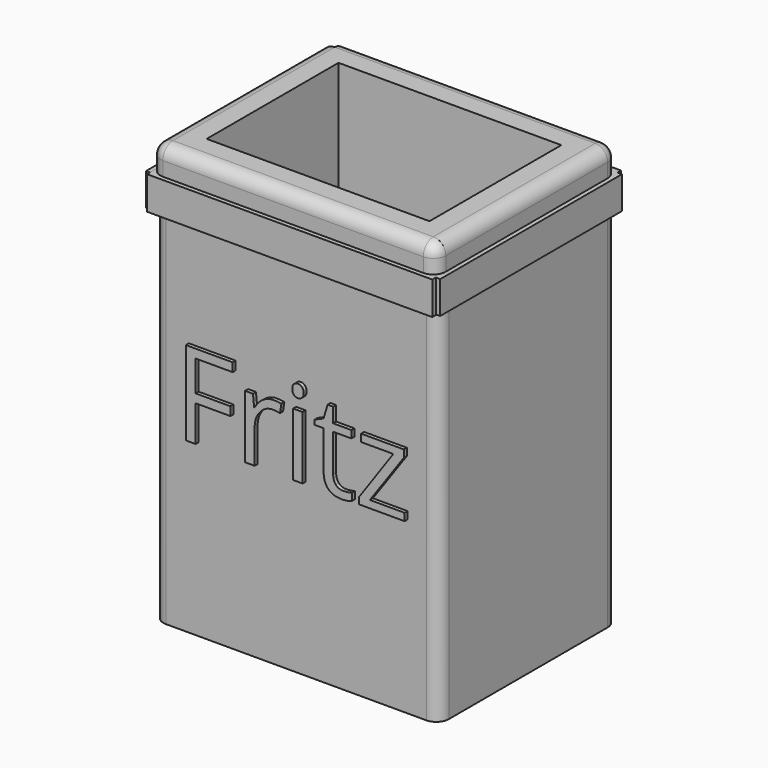
from build123d import *

# Parameters (mm, degrees)
F0_W          = 115.9102246165
F0_H          = 92.3246163875
F1_DEPTH      = 171.45
F2_T          = -12.7
F3_R          = 5.08
F4_W          = 115.9102246165
F4_H          = 13.2569223642
F6_DEPTH      = 1.778
F5_W          = 92.3246163875
F5_H          = 13.2491886616
F7_DEPTH      = 1.778
F8_W          = 92.3246163875
F8_H          = 13.2032483816
F9_DEPTH      = 1.778
F11_DEPTH     = 1.778
F12_W         = 115.9102246165
F12_H         = 147.1718251705
F12_W_2       = 3.8736611168
F12_H_2       = 25.5631778903
F13_DEPTH     = 1.524
F14_R         = 5.08
F15_T1_DEPTH  = 5.7646141005
F15_S5_W      = 5.08
F15_S5_H      = 5.08
F15_T6_DEPTH  = 5.08
F15_S11_W     = 5.08
F15_S11_H     = 5.08
F15_T12_DEPTH = 5.08
F15_S17_W     = 5.08
F15_S17_H     = 5.08
F15_T18_DEPTH = 5.08
F15_S23_W     = 5.08
F15_S23_H     = 5.08
F15_T24_DEPTH = 5.08


# Not quite as in the source:
# - a fillet or chamfer that OpenCascade refuses, or shapes differently, is made with other operations: its cross-section is extruded or revolved along the edge and cut away or added
# - a feature names something its author has since deleted; it is built from what else it names


with BuildPart() as f1:
    # F0 (on Top) → F1 (new body)
    with BuildSketch(Plane.XY):
        with Locations((2.3365281522, -22.1691494808)):
            Rectangle(F0_W, F0_H)
    extrude(amount=F1_DEPTH)

    # F2
    f2_openings = [f1.faces().sort_by_distance(p)[0] for p in [
        (2.336528, -22.169149, 171.45),
    ]]
    offset(amount=F2_T, openings=f2_openings)

    # F3
    f3_edges = [f1.edges().sort_by_distance(p)[0] for p in [
        (60.29164, -22.169149, 171.45),
        (2.336528, 23.993159, 171.45),
        (-55.618584, -22.169149, 171.45),
        (2.336528, -68.331458, 171.45),
    ]]
    fillet(f3_edges, radius=F3_R)

    # F4 (on face) → F6 (join)
    with BuildSketch(Plane(origin=(0, 23.993158713, 0), x_dir=(-1, 0, 0), z_dir=(0, 1, 0))):
        with Locations((-2.3365281522, 153.9769247174)):
            Rectangle(F4_W, F4_H)
    extrude(amount=F6_DEPTH)

    # F5 (on face) → F7 (join)
    with BuildSketch(Plane(origin=(-55.618584156, 0, 0), x_dir=(0, -1, 0), z_dir=(-1, 0, 0))):
        with Locations((22.1691494808, 153.7964195013)):
            Rectangle(F5_W, F5_H)
    extrude(amount=F7_DEPTH)

    # F8 (on face) → F9 (join)
    with BuildSketch(Plane.YZ.offset(60.2916404605)):
        with Locations((-22.1691494808, 154.0037617087)):
            Rectangle(F8_W, F8_H)
    extrude(amount=F9_DEPTH)

    # F10 (on face) → F11 (join)
    with BuildSketch(Plane.XZ.offset(68.3314576745)):
        Polygon((60.2916404605, 147.4021375179), (60.2916404605, 160.6053858995), (-55.618584156, 160.6053858995), (-55.618584156, 160.4210138321), (-55.618584156, 147.1718251705), (60.2916404605, 147.1718251705), align=None)
    extrude(amount=F11_DEPTH)

    # F12 (on face) → F13 (cut)
    with BuildSketch(Plane.XZ.offset(68.3314576745)):
        with Locations((2.3365281522, 73.5859125853)):
            Rectangle(F12_W, F12_H)
        Polygon((-37.2516920373, 83.9250860008), (-37.2516920373, 69.3484768271), (-41.214917573, 69.3484768271), (-41.214917573, 103.4501293179), (-22.2048696645, 103.4501293179), (-22.2048696645, 99.9272621751), (-37.2516920373, 99.9272621751), (-37.2516920373, 87.4479531437), (-23.1154412565, 87.4479531437), (-23.1154412565, 83.9250860008), align=None, mode=Mode.SUBTRACT)
        with BuildLine():
            add(Edge.make_bspline(
                [(-9.8897620677, 94.027206081), (-7.8820263443, 95.3818679166), (-5.4787144375, 95.3818679166)],
                knots=[0, 0, 0, 1, 1, 1], degree=2))
            add(Edge.make_bspline(
                [(-5.4787144375, 95.3818679166), (-3.7769904787, 95.3818679166), (-2.4260604938, 95.0982472568)],
                knots=[0, 0, 0, 1, 1, 1], degree=2))
            Line((-2.4260604938, 95.0982472568), (-2.9634470072, 91.5082067998))
            add(Edge.make_bspline(
                [(-2.9634470072, 91.5082067998), (-4.5457517408, 91.8590007738), (-5.7623350973, 91.8590007738)],
                knots=[0, 0, 0, 1, 1, 1], degree=2))
            add(Edge.make_bspline(
                [(-5.7623350973, 91.8590007738), (-8.867234952, 91.8590007738), (-11.0690269163, 89.3400014926)],
                knots=[0, 0, 0, 1, 1, 1], degree=2))
            add(Edge.make_bspline(
                [(-11.0690269163, 89.3400014926), (-13.2708188806, 86.8210022115), (-13.2708188806, 83.0667603198)],
                knots=[0, 0, 0, 1, 1, 1], degree=2))
            Line((-13.2708188806, 83.0667603198), (-13.2708188806, 69.3484768271))
            Line((-13.2708188806, 69.3484768271), (-17.1444799974, 69.3484768271))
            Line((-17.1444799974, 69.3484768271), (-17.1444799974, 94.9116547175))
            Line((-17.1444799974, 94.9116547175), (-13.9500157238, 94.9116547175))
            Line((-13.9500157238, 94.9116547175), (-13.5021936294, 90.1796679197))
            Line((-13.5021936294, 90.1796679197), (-13.31560109, 90.1796679197))
            add(Edge.make_bspline(
                [(-13.31560109, 90.1796679197), (-11.897497791, 92.6725442453), (-9.8897620677, 94.027206081)],
                knots=[0, 0, 0, 1, 1, 1], degree=2))
        make_face(mode=Mode.SUBTRACT)
        with Locations((4.2950027734, 82.1300657723)):
            Rectangle(F12_W_2, F12_H_2, mode=Mode.SUBTRACT)
        with BuildLine():
            add(Edge.make_bspline(
                [(19.6888872694, 73.3154342136), (20.7860514007, 72.0801916032), (22.6967590036, 72.0801916032)],
                knots=[0, 0, 0, 1, 1, 1], degree=2))
            add(Edge.make_bspline(
                [(22.6967590036, 72.0801916032), (23.7267498208, 72.0801916032), (24.6821036223, 72.2294656346)],
                knots=[0, 0, 0, 1, 1, 1], degree=2))
            add(Edge.make_bspline(
                [(24.6821036223, 72.2294656346), (25.6374574237, 72.3787396661), (26.1972350418, 72.5429411007)],
                knots=[0, 0, 0, 1, 1, 1], degree=2))
            Line((26.1972350418, 72.5429411007), (26.1972350418, 69.5798515759))
            add(Edge.make_bspline(
                [(26.1972350418, 69.5798515759), (25.5702841096, 69.281303513), (24.3462370515, 69.0797835705)],
                knots=[0, 0, 0, 1, 1, 1], degree=2))
            add(Edge.make_bspline(
                [(24.3462370515, 69.0797835705), (23.1221899933, 68.878263628), (22.1369813856, 68.878263628)],
                knots=[0, 0, 0, 1, 1, 1], degree=2))
            add(Edge.make_bspline(
                [(22.1369813856, 68.878263628), (14.7255257228, 68.878263628), (14.7255257228, 76.6927591758)],
                knots=[0, 0, 0, 1, 1, 1], degree=2))
            Line((14.7255257228, 76.6927591758), (14.7255257228, 91.9037829832))
            Line((14.7255257228, 91.9037829832), (11.0608482501, 91.9037829832))
            Line((11.0608482501, 91.9037829832), (11.0608482501, 93.7697083767))
            Line((11.0608482501, 93.7697083767), (14.7255257228, 95.3818679166))
            Line((14.7255257228, 95.3818679166), (16.3526126659, 100.8378337671))
            Line((16.3526126659, 100.8378337671), (18.591723138, 100.8378337671))
            Line((18.591723138, 100.8378337671), (18.591723138, 94.9116547175))
            Line((18.591723138, 94.9116547175), (26.0106425024, 94.9116547175))
            Line((26.0106425024, 94.9116547175), (26.0106425024, 91.9037829832))
            Line((26.0106425024, 91.9037829832), (18.591723138, 91.9037829832))
            Line((18.591723138, 91.9037829832), (18.591723138, 76.8569606104))
            add(Edge.make_bspline(
                [(18.591723138, 76.8569606104), (18.591723138, 74.5506768241), (19.6888872694, 73.3154342136)],
                knots=[0, 0, 0, 1, 1, 1], degree=2))
        make_face(mode=Mode.SUBTRACT)
        with BuildLine():
            add(Edge.make_bspline(
                [(2.6828432334, 99.8899436672), (2.0297693457, 100.5318220026), (2.0297693457, 101.837969778)],
                knots=[0, 0, 0, 1, 1, 1], degree=2))
            add(Edge.make_bspline(
                [(2.0297693457, 101.837969778), (2.0297693457, 103.1665086581), (2.6828432334, 103.7859958888)],
                knots=[0, 0, 0, 1, 1, 1], degree=2))
            add(Edge.make_bspline(
                [(2.6828432334, 103.7859958888), (3.3359171211, 104.4054831194), (4.3211257289, 104.4054831194)],
                knots=[0, 0, 0, 1, 1, 1], degree=2))
            add(Edge.make_bspline(
                [(4.3211257289, 104.4054831194), (5.2540884256, 104.4054831194), (5.9295534181, 103.7748003364)],
                knots=[0, 0, 0, 1, 1, 1], degree=2))
            add(Edge.make_bspline(
                [(5.9295534181, 103.7748003364), (6.6050184105, 103.1441175534), (6.6050184105, 101.837969778)],
                knots=[0, 0, 0, 1, 1, 1], degree=2))
            add(Edge.make_bspline(
                [(6.6050184105, 101.837969778), (6.6050184105, 100.5318220026), (5.9295534181, 99.8899436672)],
                knots=[0, 0, 0, 1, 1, 1], degree=2))
            add(Edge.make_bspline(
                [(5.9295534181, 99.8899436672), (5.2540884256, 99.2480653319), (4.3211257289, 99.2480653319)],
                knots=[0, 0, 0, 1, 1, 1], degree=2))
            add(Edge.make_bspline(
                [(4.3211257289, 99.2480653319), (3.3359171211, 99.2480653319), (2.6828432334, 99.8899436672)],
                knots=[0, 0, 0, 1, 1, 1], degree=2))
        make_face(mode=Mode.SUBTRACT)
        Polygon((47.6553770665, 72.3563485614), (47.6553770665, 69.3484768271), (29.1080786556, 69.3484768271), (29.1080786556, 71.9831634827), (43.057736897, 91.9037829832), (29.9738680381, 91.9037829832), (29.9738680381, 94.9116547175), (47.3045830925, 94.9116547175), (47.3045830925, 91.9037829832), (33.5415173904, 72.3563485614), align=None, mode=Mode.SUBTRACT)
    extrude(amount=-F13_DEPTH, mode=Mode.SUBTRACT)

    # F14
    f14_edges = [f1.edges().sort_by_distance(p)[0] for p in [
        (60.29164, -66.807458, 73.585913),
        (-55.618584, -66.807458, 73.585913),
        (-55.618584, 23.993159, 73.585913),
        (60.29164, 23.993159, 73.674232),
    ]]
    fillet(f14_edges, radius=F14_R)

    # F15: fillet of radius 5.08 on 4 edges, made by hand

    # F15_s2 → F15_t1 (cut)
    with BuildSketch(Plane.XY.offset(160.6053858995)):
        with BuildLine():
            ThreePointArc((-55.618584156, -63.2514576745), (-54.1306866045, -66.8435601229), (-50.538584156, -68.3314576745))
            Line((-50.538584156, -68.3314576745), (-55.618584156, -68.3314576745))
            Line((-55.618584156, -68.3314576745), (-55.618584156, -63.2514576745))
        make_face()
        with BuildLine():
            ThreePointArc((55.2116404605, -68.3314576745), (58.8037429089, -66.8435601229), (60.2916404605, -63.2514576745))
            Line((60.2916404605, -63.2514576745), (60.2916404605, -68.3314576745))
            Line((60.2916404605, -68.3314576745), (55.2116404605, -68.3314576745))
        make_face()
        with BuildLine():
            ThreePointArc((55.2116404605, 23.993158713), (58.8037429089, 22.5052611614), (60.2916404605, 18.913158713))
            Line((60.2916404605, 18.913158713), (60.2916404605, 23.993158713))
            Line((60.2916404605, 23.993158713), (55.2116404605, 23.993158713))
        make_face()
        with BuildLine():
            ThreePointArc((-55.618584156, 18.913158713), (-54.1306866045, 22.5052611614), (-50.538584156, 23.993158713))
            Line((-50.538584156, 23.993158713), (-55.618584156, 23.993158713))
            Line((-55.618584156, 23.993158713), (-55.618584156, 18.913158713))
        make_face()
    extrude(amount=F15_T1_DEPTH, mode=Mode.SUBTRACT)


with BuildPart() as f15_tool4:
    # F15_s5 → F15_t6 (new body)
    with BuildSketch(Plane.YZ.offset(-50.538584156)):
        with Locations((21.453158713, 168.91)):
            Rectangle(F15_S5_W, F15_S5_H)
    extrude(amount=-F15_T6_DEPTH)

    # F15_s7 → F15_t8 (revolve, cut)
    with BuildSketch(Plane(origin=(-50.538584156, 18.913158713, 166.37), x_dir=(0, -0.7071067812, -0.7071067812), z_dir=(0, 0.7071067812, -0.7071067812))):
        with BuildLine():
            ThreePointArc((0, -5.08), (5.08, 0), (0, 5.08))
            Line((0, 5.08), (0, -5.08))
        make_face()
    revolve(axis=Axis((-50.538584156, 18.913158713, 166.37), (-1, 0, 0)), mode=Mode.SUBTRACT)


with BuildPart() as f1_1:
    add(f1.part)

    # F15_t3: cut F15_tool4
    add(f15_tool4.part, mode=Mode.SUBTRACT)


with BuildPart() as f15_tool10:
    # F15_s11 → F15_t12 (new body)
    with BuildSketch(Plane.XZ.offset(-18.913158713)):
        with Locations((57.7516404605, 168.91)):
            Rectangle(F15_S11_W, F15_S11_H)
    extrude(amount=-F15_T12_DEPTH)

    # F15_s13 → F15_t14 (revolve, cut)
    with BuildSketch(Plane(origin=(55.2116404605, 18.913158713, 166.37), x_dir=(-0.7071067812, 0, -0.7071067812), z_dir=(0.7071067812, 0, -0.7071067812))):
        with BuildLine():
            ThreePointArc((0, -5.08), (5.08, 0), (0, 5.08))
            Line((0, 5.08), (0, -5.08))
        make_face()
    revolve(axis=Axis((55.2116404605, 18.913158713, 166.37), (0, 1, 0)), mode=Mode.SUBTRACT)


with BuildPart() as f1_2:
    add(f1_1.part)

    # F15_t9: cut F15_tool10
    add(f15_tool10.part, mode=Mode.SUBTRACT)


with BuildPart() as f15_tool16:
    # F15_s17 → F15_t18 (new body)
    with BuildSketch(Plane.XZ.offset(63.2514576745)):
        with Locations((57.7516404605, 168.91)):
            Rectangle(F15_S17_W, F15_S17_H)
    extrude(amount=F15_T18_DEPTH)

    # F15_s19 → F15_t20 (revolve, cut)
    with BuildSketch(Plane(origin=(55.2116404605, -63.2514576745, 166.37), x_dir=(-0.7071067812, 0, -0.7071067812), z_dir=(-0.7071067812, 0, 0.7071067812))):
        with BuildLine():
            ThreePointArc((0, -5.08), (5.08, 0), (0, 5.08))
            Line((0, 5.08), (0, -5.08))
        make_face()
    revolve(axis=Axis((55.2116404605, -63.2514576745, 166.37), (0, -1, 0)), mode=Mode.SUBTRACT)


with BuildPart() as f1_3:
    add(f1_2.part)

    # F15_t15: cut F15_tool16
    add(f15_tool16.part, mode=Mode.SUBTRACT)


with BuildPart() as f15_tool22:
    # F15_s23 → F15_t24 (new body)
    with BuildSketch(Plane.YZ.offset(-50.538584156)):
        with Locations((-65.7914576745, 168.91)):
            Rectangle(F15_S23_W, F15_S23_H)
    extrude(amount=-F15_T24_DEPTH)

    # F15_s25 → F15_t26 (revolve, cut)
    with BuildSketch(Plane(origin=(-50.538584156, -63.2514576745, 166.37), x_dir=(0, 0.7071067812, -0.7071067812), z_dir=(0, 0.7071067812, 0.7071067812))):
        with BuildLine():
            ThreePointArc((0, -5.08), (5.08, 0), (0, 5.08))
            Line((0, 5.08), (0, -5.08))
        make_face()
    revolve(axis=Axis((-50.538584156, -63.2514576745, 166.37), (-1, 0, 0)), mode=Mode.SUBTRACT)


with BuildPart() as f1_4:
    add(f1_3.part)

    # F15_t21: cut F15_tool22
    add(f15_tool22.part, mode=Mode.SUBTRACT)


solid = f1_4.part
